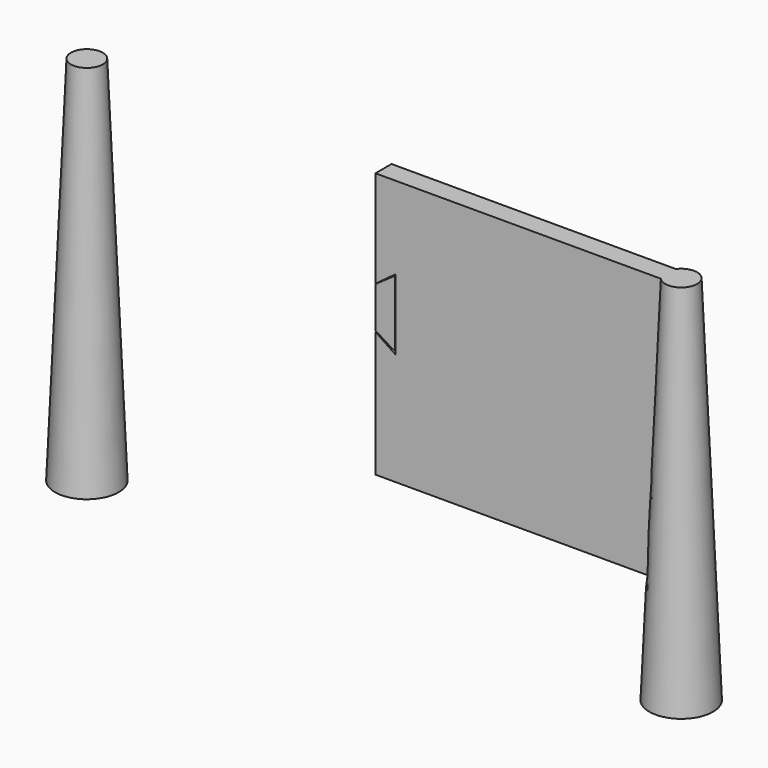
from build123d import *

# Parameters (mm, degrees)
F0_R      = 3
F2_R      = 1.5
F4_W      = 27
F4_H      = 1.8959337356
F5_DEPTH  = 25
F7_R      = 1.5
F6_R      = 3
F13_DEPTH = 25
F15_DEPTH = 2


with BuildPart() as f3:
    # F0 (on Top) → F3 section 0
    with BuildSketch(Plane.XY):
        with Locations((28, 0)):
            Circle(F0_R)
    # F2 (on offset) → F3 section 1
    with BuildSketch(Plane.XY.offset(35)):
        with Locations((28, 0)):
            Circle(F2_R)
    loft()

    # F4 (on offset) → F5 (join)
    with BuildSketch(Plane.XY.offset(35)):
        with Locations((13.5, -0.0643532243)):
            Rectangle(F4_W, F4_H)
    extrude(amount=-F5_DEPTH)

    # F12 (on face) → F13 (cut)
    with BuildSketch(Plane.XZ.offset(1.0123200921)):
        Polygon((1.8713724567, 27.2230319679), (0, 25.8460454643), (0, 21.8402631581), (1.8713724567, 20.5884557217), align=None)
    extrude(amount=-F13_DEPTH, mode=Mode.SUBTRACT)


with BuildPart() as f8:
    # F7 (on offset) → F8 section 0
    with BuildSketch(Plane.XY.offset(35)):
        with Locations((-28, 0)):
            Circle(F7_R)
    # F6 (on Top) → F8 section 1
    with BuildSketch(Plane.XY):
        with Locations((-28, 0)):
            Circle(F6_R)
    loft()


with BuildPart() as f15:
    # F14 (on face) → F15 (new body)
    with BuildSketch(Plane(origin=(0, -1.0163254858, 0), x_dir=(-1, 0, 0), z_dir=(0, 1, 0))):
        Polygon((0, 21.9585560262), (0, 25.8090086281), (-1.8292188179, 27.0924922079), (-1.8292188179, 20.829975605), align=None)
    extrude(amount=F15_DEPTH)


solid = Compound([f3.part, f8.part, f15.part])
